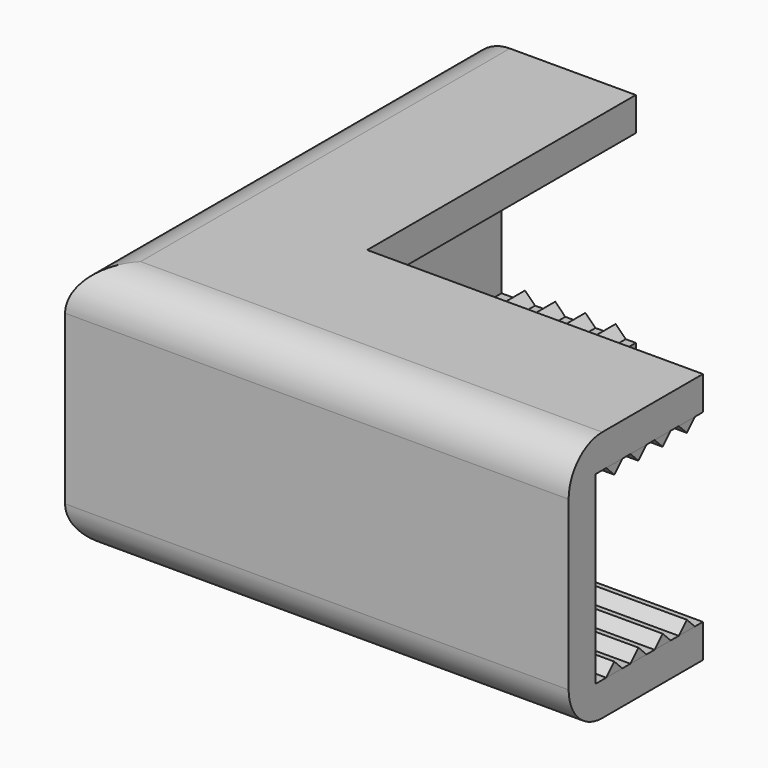
from build123d import *

# Parameters (mm, degrees)
F1_DEPTH   = 38.1
F2_T       = -5.08
F3_R       = 6.35
F4_R       = 6.35
F5_W       = 50.8
F5_H       = 3.048
F6_DEPTH   = 1.524
F5_R       = 3.175
F5_W_2     = 3.048
F5_H_2     = 50.8
F7_SIZE    = 1.52399
F7_2_SIZE  = 1.52399
F7_3_SIZE  = 1.52399
F7_4_SIZE  = 1.52399
F7_5_SIZE  = 1.52399
F7_6_SIZE  = 1.52399
F7_7_SIZE  = 1.52399
F7_8_SIZE  = 1.52399
F7_9_SIZE  = 1.52399
F7_10_SIZE = 1.52399
F7_11_SIZE = 1.52399
F7_12_SIZE = 1.52399
F8_T       = -0.508


# Not quite as in the source:
# - a fillet or chamfer is up to 0.001 mm smaller than in the source, because OpenCascade refuses the exact size


with BuildPart() as f1:
    # F0 (on Top) → F1 (new body)
    with BuildSketch(Plane.XY):
        Polygon((-23.7132772938, 50.8), (-49.1132772938, 50.8), (-49.1132772938, -25.4), (27.0867227062, -25.4), (27.0867227062, 0), (-23.7132772938, 0), align=None)
    extrude(amount=F1_DEPTH)

    # F2
    f2_openings = [f1.faces().sort_by_distance(p)[0] for p in [
        (1.686723, 0, 19.05),
        (-23.713277, 25.4, 19.05),
        (27.086723, -12.7, 19.05),
        (-36.413277, 50.8, 19.05),
    ]]
    offset(amount=F2_T, openings=f2_openings)

    # F3
    f3_edges = [f1.edges().sort_by_distance(p)[0] for p in [
        (-11.013277, -25.4, 38.1),
        (-49.113277, 12.7, 38.1),
    ]]
    fillet(f3_edges, radius=F3_R)

    # F4
    f4_edges = [f1.edges().sort_by_distance(p)[0] for p in [
        (-49.113277, 12.7, 0),
        (-11.013277, -25.4, 0),
    ]]
    fillet(f4_edges, radius=F4_R)


with BuildPart() as f6:
    # F5 (on face) → F6 (new body)
    with BuildSketch(Plane.XY.offset(5.08)):
        with Locations((1.6867227062, -3.048)):
            Rectangle(F5_W, F5_H)
    extrude(amount=F6_DEPTH)

    # F7#8 (size 1.524 in the source; OpenCascade refuses exactly that, so slightly less here)
    f7_8_edges = [f6.edges().sort_by_distance(p)[0] for p in [
        (1.686723, -4.572, 6.604),
        (1.686723, -1.524, 6.604),
    ]]
    chamfer(f7_8_edges, length=F7_8_SIZE)

    # F8 (hollow: no face is removed)
    offset(amount=F8_T, mode=Mode.SUBTRACT)


with BuildPart() as f6b:
    # F5 (on face) → F6, piece 2 (new body)
    with BuildSketch(Plane.XY.offset(5.08)):
        with Locations((1.6867227062, -7.62)):
            Rectangle(F5_W, F5_H)
    extrude(amount=F6_DEPTH)

    # F7#7 (size 1.524 in the source; OpenCascade refuses exactly that, so slightly less here)
    f7_7_edges = [f6b.edges().sort_by_distance(p)[0] for p in [
        (1.686723, -9.144, 6.604),
        (1.686723, -6.096, 6.604),
    ]]
    chamfer(f7_7_edges, length=F7_7_SIZE)

    # F8#6 (hollow: no face is removed)
    offset(amount=F8_T, mode=Mode.SUBTRACT)


with BuildPart() as f6c:
    # F5 (on face) → F6, piece 3 (new body)
    with BuildSketch(Plane.XY.offset(5.08)):
        with Locations((1.6867227062, -12.192)):
            Rectangle(F5_W, F5_H)
    extrude(amount=F6_DEPTH)

    # F7#6 (size 1.524 in the source; OpenCascade refuses exactly that, so slightly less here)
    f7_6_edges = [f6c.edges().sort_by_distance(p)[0] for p in [
        (1.686723, -13.716, 6.604),
        (1.686723, -10.668, 6.604),
    ]]
    chamfer(f7_6_edges, length=F7_6_SIZE)

    # F8#7 (hollow: no face is removed)
    offset(amount=F8_T, mode=Mode.SUBTRACT)


with BuildPart() as f6d:
    # F5 (on face) → F6, piece 4 (new body)
    with BuildSketch(Plane.XY.offset(5.08)):
        with Locations((1.6867227062, -16.764)):
            Rectangle(F5_W, F5_H)
    extrude(amount=F6_DEPTH)

    # F7#5 (size 1.524 in the source; OpenCascade refuses exactly that, so slightly less here)
    f7_5_edges = [f6d.edges().sort_by_distance(p)[0] for p in [
        (1.686723, -18.288, 6.604),
        (1.686723, -15.24, 6.604),
    ]]
    chamfer(f7_5_edges, length=F7_5_SIZE)

    # F8#8 (hollow: no face is removed)
    offset(amount=F8_T, mode=Mode.SUBTRACT)


with BuildPart() as f6e:
    # F5 (on face) → F6, piece 5 (new body)
    with BuildSketch(Plane.XY.offset(5.08)):
        with Locations((-38.0007772938, -14.2875)):
            Circle(F5_R)
    extrude(amount=F6_DEPTH)

    # F7#3 (size 1.524 in the source; OpenCascade refuses exactly that, so slightly less here)
    f7_3_edges = [f6e.edges().sort_by_distance(p)[0] for p in [
        (-41.175777, -14.2875, 6.604),
    ]]
    chamfer(f7_3_edges, length=F7_3_SIZE)

    # F8#3 (hollow: no face is removed)
    offset(amount=F8_T, mode=Mode.SUBTRACT)


with BuildPart() as f6f:
    # F5 (on face) → F6, piece 6 (new body)
    with BuildSketch(Plane.XY.offset(5.08)):
        with Locations((-40.4772772938, 25.4)):
            Rectangle(F5_W_2, F5_H_2)
    extrude(amount=F6_DEPTH)

    # F7#12 (size 1.524 in the source; OpenCascade refuses exactly that, so slightly less here)
    f7_12_edges = [f6f.edges().sort_by_distance(p)[0] for p in [
        (-38.953277, 25.4, 6.604),
        (-42.001277, 25.4, 6.604),
    ]]
    chamfer(f7_12_edges, length=F7_12_SIZE)

    # F8#12 (hollow: no face is removed)
    offset(amount=F8_T, mode=Mode.SUBTRACT)


with BuildPart() as f6g:
    # F5 (on face) → F6, piece 7 (new body)
    with BuildSketch(Plane.XY.offset(5.08)):
        with Locations((-35.9052772938, 25.4)):
            Rectangle(F5_W_2, F5_H_2)
    extrude(amount=F6_DEPTH)

    # F7#11 (size 1.524 in the source; OpenCascade refuses exactly that, so slightly less here)
    f7_11_edges = [f6g.edges().sort_by_distance(p)[0] for p in [
        (-34.381277, 25.4, 6.604),
        (-37.429277, 25.4, 6.604),
    ]]
    chamfer(f7_11_edges, length=F7_11_SIZE)

    # F8#11 (hollow: no face is removed)
    offset(amount=F8_T, mode=Mode.SUBTRACT)


with BuildPart() as f6h:
    # F5 (on face) → F6, piece 8 (new body)
    with BuildSketch(Plane.XY.offset(5.08)):
        with Locations((-31.3332772938, 25.4)):
            Rectangle(F5_W_2, F5_H_2)
    extrude(amount=F6_DEPTH)

    # F7#10 (size 1.524 in the source; OpenCascade refuses exactly that, so slightly less here)
    f7_10_edges = [f6h.edges().sort_by_distance(p)[0] for p in [
        (-29.809277, 25.4, 6.604),
        (-32.857277, 25.4, 6.604),
    ]]
    chamfer(f7_10_edges, length=F7_10_SIZE)

    # F8#10 (hollow: no face is removed)
    offset(amount=F8_T, mode=Mode.SUBTRACT)


with BuildPart() as f6i:
    # F5 (on face) → F6, piece 9 (new body)
    with BuildSketch(Plane.XY.offset(5.08)):
        with Locations((-26.7612772938, 25.4)):
            Rectangle(F5_W_2, F5_H_2)
    extrude(amount=F6_DEPTH)

    # F7#9 (size 1.524 in the source; OpenCascade refuses exactly that, so slightly less here)
    f7_9_edges = [f6i.edges().sort_by_distance(p)[0] for p in [
        (-25.237277, 25.4, 6.604),
        (-28.285277, 25.4, 6.604),
    ]]
    chamfer(f7_9_edges, length=F7_9_SIZE)

    # F8#9 (hollow: no face is removed)
    offset(amount=F8_T, mode=Mode.SUBTRACT)


with BuildPart() as f6j:
    # F5 (on face) → F6, piece 10 (new body)
    with BuildSketch(Plane.XY.offset(5.08)):
        with Locations((-28.4757772938, -4.7625)):
            Circle(F5_R)
    extrude(amount=F6_DEPTH)

    # F7#2 (size 1.524 in the source; OpenCascade refuses exactly that, so slightly less here)
    f7_2_edges = [f6j.edges().sort_by_distance(p)[0] for p in [
        (-31.650777, -4.7625, 6.604),
    ]]
    chamfer(f7_2_edges, length=F7_2_SIZE)

    # F8#5 (hollow: no face is removed)
    offset(amount=F8_T, mode=Mode.SUBTRACT)


with BuildPart() as f6k:
    # F5 (on face) → F6, piece 11 (new body)
    with BuildSketch(Plane.XY.offset(5.08)):
        with Locations((-38.0007772938, -4.7625)):
            Circle(F5_R)
    extrude(amount=F6_DEPTH)

    # F7 (size 1.524 in the source; OpenCascade refuses exactly that, so slightly less here)
    f7_edges = [f6k.edges().sort_by_distance(p)[0] for p in [
        (-41.175777, -4.7625, 6.604),
    ]]
    chamfer(f7_edges, length=F7_SIZE)

    # F8#4 (hollow: no face is removed)
    offset(amount=F8_T, mode=Mode.SUBTRACT)


with BuildPart() as f6l:
    # F5 (on face) → F6, piece 12 (new body)
    with BuildSketch(Plane.XY.offset(5.08)):
        with Locations((-28.4757772938, -14.2875)):
            Circle(F5_R)
    extrude(amount=F6_DEPTH)

    # F7#4 (size 1.524 in the source; OpenCascade refuses exactly that, so slightly less here)
    f7_4_edges = [f6l.edges().sort_by_distance(p)[0] for p in [
        (-31.650777, -14.2875, 6.604),
    ]]
    chamfer(f7_4_edges, length=F7_4_SIZE)

    # F8#2 (hollow: no face is removed)
    offset(amount=F8_T, mode=Mode.SUBTRACT)


with BuildPart() as f13_1:
    # F13: instance of F1
    add(f1.part.mirror(Plane(origin=(27.0867227062, -25.4, 19.05), x_dir=(-0.6823182504, 0.7310552682, 0), z_dir=(0, 0, -1))))


with BuildPart() as f13_2:
    # F13: instance of F6
    add(f6.part.mirror(Plane(origin=(27.0867227062, -25.4, 19.05), x_dir=(-0.6823182504, 0.7310552682, 0), z_dir=(0, 0, -1))))


with BuildPart() as f13_3:
    # F13: instance of F6i
    add(f6i.part.mirror(Plane(origin=(27.0867227062, -25.4, 19.05), x_dir=(-0.6823182504, 0.7310552682, 0), z_dir=(0, 0, -1))))


with BuildPart() as f13_4:
    # F13: instance of F6j
    add(f6j.part.mirror(Plane(origin=(27.0867227062, -25.4, 19.05), x_dir=(-0.6823182504, 0.7310552682, 0), z_dir=(0, 0, -1))))


with BuildPart() as f13_5:
    # F13: instance of F6l
    add(f6l.part.mirror(Plane(origin=(27.0867227062, -25.4, 19.05), x_dir=(-0.6823182504, 0.7310552682, 0), z_dir=(0, 0, -1))))


with BuildPart() as f13_6:
    # F13: instance of F6d
    add(f6d.part.mirror(Plane(origin=(27.0867227062, -25.4, 19.05), x_dir=(-0.6823182504, 0.7310552682, 0), z_dir=(0, 0, -1))))


with BuildPart() as f13_7:
    # F13: instance of F6c
    add(f6c.part.mirror(Plane(origin=(27.0867227062, -25.4, 19.05), x_dir=(-0.6823182504, 0.7310552682, 0), z_dir=(0, 0, -1))))


with BuildPart() as f13_8:
    # F13: instance of F6b
    add(f6b.part.mirror(Plane(origin=(27.0867227062, -25.4, 19.05), x_dir=(-0.6823182504, 0.7310552682, 0), z_dir=(0, 0, -1))))


with BuildPart() as f13_9:
    # F13: instance of F6e
    add(f6e.part.mirror(Plane(origin=(27.0867227062, -25.4, 19.05), x_dir=(-0.6823182504, 0.7310552682, 0), z_dir=(0, 0, -1))))


with BuildPart() as f13_10:
    # F13: instance of F6k
    add(f6k.part.mirror(Plane(origin=(27.0867227062, -25.4, 19.05), x_dir=(-0.6823182504, 0.7310552682, 0), z_dir=(0, 0, -1))))


with BuildPart() as f13_11:
    # F13: instance of F6h
    add(f6h.part.mirror(Plane(origin=(27.0867227062, -25.4, 19.05), x_dir=(-0.6823182504, 0.7310552682, 0), z_dir=(0, 0, -1))))


with BuildPart() as f13_12:
    # F13: instance of F6g
    add(f6g.part.mirror(Plane(origin=(27.0867227062, -25.4, 19.05), x_dir=(-0.6823182504, 0.7310552682, 0), z_dir=(0, 0, -1))))


with BuildPart() as f13_13:
    # F13: instance of F6f
    add(f6f.part.mirror(Plane(origin=(27.0867227062, -25.4, 19.05), x_dir=(-0.6823182504, 0.7310552682, 0), z_dir=(0, 0, -1))))


solid = Compound([f1.part, f6.part, f6b.part, f6c.part, f6d.part, f6e.part, f6f.part, f6g.part, f6h.part, f6i.part, f6j.part, f6k.part, f6l.part, f13_1.part, f13_2.part, f13_3.part, f13_4.part, f13_5.part, f13_6.part, f13_7.part, f13_8.part, f13_9.part, f13_10.part, f13_11.part, f13_12.part, f13_13.part])
